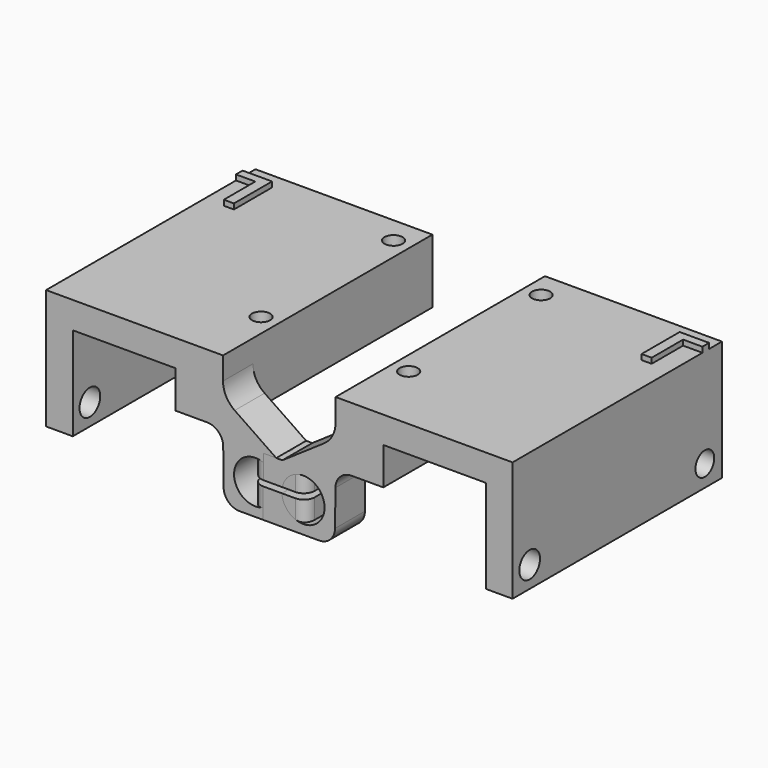
from build123d import *

# Parameters (mm, degrees)
F1_DEPTH      = 7
F2_DEPTH      = 42
F3_R          = 1.7
F3_R_2        = 11
F4_DEPTH      = 12.001
F5_R          = 4
F6_DEPTH      = 10
F7_DEPTH      = 12.001
F8_R          = 1.4
F9_DEPTH      = 10.9920075553
F8_R_2        = 1.7
F10_DEPTH     = 4.4348209087
F11_R         = 5
F12_R         = 3
F13_R         = 3
F14_R         = 2
F15_R         = 2.2
F15_R_2       = 2.4255023423
F16_DEPTH     = 6
F17_TEXT_SIZE = 12.5
F18_DEPTH     = 1


# Not quite as in the source:
# - a feature names something its author has since deleted; it is built from what else it names
# - Text() gives the source's letters only with a copy of the font that has no kerning and outlines rounded to 1/6400 em; it was checked with that copy


with BuildPart() as f1:
    # F0 (on Front) → F1 (new body)
    with BuildSketch(Plane.XZ):
        Polygon((-18.6721007523, 29.8099789735), (-18.6721007523, 7.3259699669), (-13.6721007523, 7.3259699669), (-13.6721007523, 24.8099789735), (5.5278992477, 24.8099789735), (5.5278992477, 17.8099789735), (14.4637966118, 17.8099789735), (14.4637966118, 22.9406704692), (14.4637966118, 29.8099789735), align=None)
        Polygon((24.4301751077, 16.1394868046), (14.4637966118, 22.9406704692), (14.4637966118, 17.8099789735), (14.5940201178, 5.1484792493), (30.0186601057, 5.1484792493), (30.0186601057, 10.6682249423), (22.6860510706, 10.6682249423), (22.6860510706, 11.7046658959), (29.9896428882, 11.7046658959), (29.9896428882, 16.1394868046), align=None)
    extrude(amount=F1_DEPTH)

    # F0 (on Front) → F2 (join)
    with BuildSketch(Plane.XZ):
        Polygon((-18.6721007523, 29.8099789735), (-18.6721007523, 7.3259699669), (-13.6721007523, 7.3259699669), (-13.6721007523, 24.8099789735), (5.5278992477, 24.8099789735), (5.5278992477, 17.8099789735), (14.4637966118, 17.8099789735), (14.4637966118, 22.9406704692), (14.4637966118, 29.8099789735), align=None)
    extrude(amount=-F2_DEPTH)

    # F3 (on face) → F4 (cut, through all)
    with BuildSketch(Plane(origin=(0, 0, 17.8099789735), x_dir=(1, 0, 0), z_dir=(0, 0, -1))):
        with Locations((11.1850741468, -6)):
            Circle(F3_R)
        with Locations((11.1850741468, -37)):
            Circle(F3_R)
        with Locations((26.6850741468, -21.5)):
            Circle(F3_R_2)
    extrude(amount=-F4_DEPTH, mode=Mode.SUBTRACT)

    # F5 (on face) → F6 (cut)
    with BuildSketch(Plane.XZ.offset(7)):
        with Locations((20.5278992477, 10.8989789735)):
            Circle(F5_R)
    extrude(amount=-F6_DEPTH, mode=Mode.SUBTRACT)

    # F3 (on face) → F7 (cut, through all)
    with BuildSketch(Plane(origin=(0, 0, 17.8099789735), x_dir=(1, 0, 0), z_dir=(0, 0, -1))):
        with Locations((11.1850741468, -6)):
            Circle(F3_R)
        with Locations((11.1850741468, -37)):
            Circle(F3_R)
        with Locations((26.6850741468, -21.5)):
            Circle(F3_R_2)
    extrude(amount=-F7_DEPTH, mode=Mode.SUBTRACT)

    # F8 (on face) → F9 (cut, through all)
    with BuildSketch(Plane.XY.offset(16.1394868046)):
        with Locations((26.9896428882, -3.5767070949)):
            Circle(F8_R)
    extrude(amount=-F9_DEPTH, mode=Mode.SUBTRACT)

    # F8 (on face) → F10 (cut, through all)
    with BuildSketch(Plane.XY.offset(16.1394868046)):
        with Locations((26.9896428882, -3.5767070949)):
            Circle(F8_R_2)
        with Locations((26.9896428882, -3.5767070949)):
            Circle(F8_R, mode=Mode.SUBTRACT)
    extrude(amount=-F10_DEPTH, mode=Mode.SUBTRACT)

    # F11
    f11_edges = [f1.edges().sort_by_distance(p)[0] for p in [
        (14.463797, -3.5, 22.94067),
    ]]
    fillet(f11_edges, radius=F11_R)

    # F12
    f12_edges = [f1.edges().sort_by_distance(p)[0] for p in [
        (14.463797, -3.5, 17.809979),
    ]]
    fillet(f12_edges, radius=F12_R)

    # F13
    f13_edges = [f1.edges().sort_by_distance(p)[0] for p in [
        (14.59402, -3.5, 5.148479),
    ]]
    fillet(f13_edges, radius=F13_R)

    # F14
    f14_edges = [f1.edges().sort_by_distance(p)[0] for p in [
        (29.989643, -7, 13.922076),
        (30.01866, -7, 7.908352),
        (29.989643, 0, 13.922076),
        (30.01866, 0, 7.908352),
    ]]
    fillet(f14_edges, radius=F14_R)

    # F15 (on face) → F16 (cut)
    with BuildSketch(Plane(origin=(-18.6721007523, 0, 0), x_dir=(0, -1, 0), z_dir=(-1, 0, 0))):
        with Locations((-38, 11.3259699669)):
            Circle(F15_R)
        with Locations((3, 11.3259699669)):
            Circle(F15_R_2)
    extrude(amount=-F16_DEPTH, mode=Mode.SUBTRACT)

    # F17 (on face) → F18 (join)
    with BuildSketch(Plane.XY.offset(29.8099789735)):
        with Locations(Location((-12.0373351273, 39), (0, 0, 180))):
            Text('L', F17_TEXT_SIZE, font='Open Sans', font_style=FontStyle.BOLD, text_align=(TextAlign.LEFT, TextAlign.BOTTOM))
    extrude(amount=F18_DEPTH)


with BuildPart() as f19_1:
    # F19: instance of F1
    add(f1.part.mirror(Plane.YZ))


with BuildPart() as f19_1_1:
    # F20: moved
    add(f19_1.part.moved(Location((50, 0, 0))))


solid = Compound([f1.part, f19_1_1.part])
